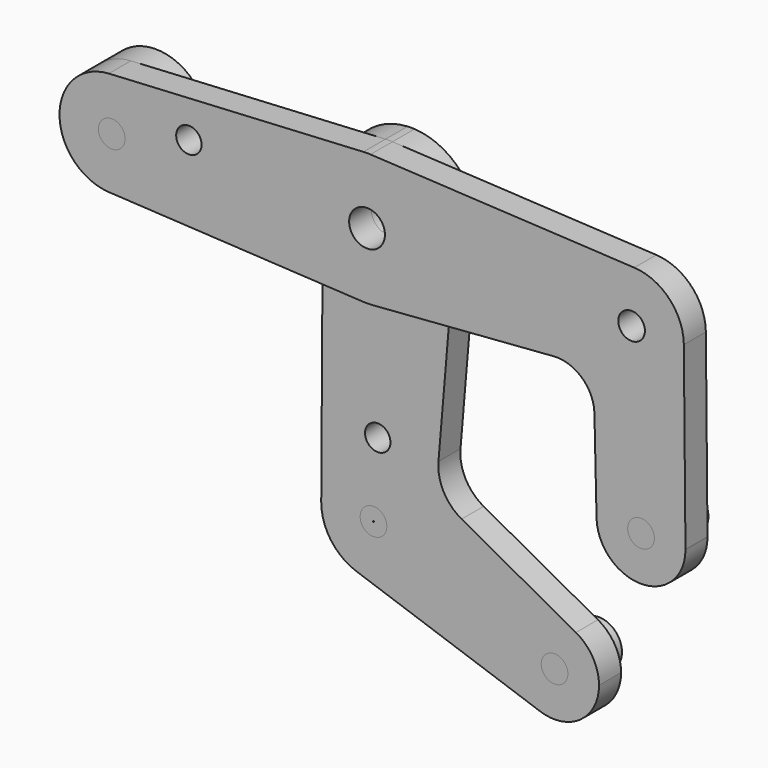
from build123d import *

# Parameters (mm, degrees)
F0_R     = 6.1493367897
F0_R_2   = 5.8576786547
F0_R_3   = 8.2510252631
F1_DEPTH = 12.7
F2_DEPTH = 12.7
F3_R     = 10.7566179169
F5_DEPTH = 25.4
F3_R_2   = 24.0961882632
F4_R     = 24.0590637796
F4_R_2   = 0.2663452523
F4_R_3   = 10.7566179169


with BuildPart() as f1:
    # F0 (on Front) → F1 (new body)
    with BuildSketch(Plane.XZ):
        with BuildLine():
            ThreePointArc((-137.004724496, 53.7728478672), (-144.5318286506, 71.2683255862), (-162.4105469667, 77.8334203262))
            ThreePointArc((-162.4105469667, 77.8334203262), (-185.1971010223, 53.7728478672), (-162.4105469667, 29.7122754082))
            ThreePointArc((-162.4105469667, 29.7122754082), (-144.5318286506, 36.2773701482), (-137.004724496, 53.7728478672))
        make_face()
        with Locations((-161.1009127591, 53.7728478672)):
            Circle(F0_R, mode=Mode.SUBTRACT)
        with BuildLine():
            ThreePointArc((-73.8970993097, 53.9616213386), (-65.4796718147, 74.8089623918), (-45.0619767979, 84.2207871257))
            Line((-45.0619767979, 84.2207871257), (-162.4105469667, 77.8334203262))
            ThreePointArc((-162.4105469667, 77.8334203262), (-144.5318286506, 71.2683255862), (-137.004724496, 53.7728478672))
            ThreePointArc((-137.004724496, 53.7728478672), (-144.5318286506, 36.2773701482), (-162.4105469667, 29.7122754082))
            Line((-162.4105469667, 29.7122754082), (-74.0769888087, 24.9042165128))
            Line((-74.0769888087, 24.9042165128), (-73.8970993097, 53.9616213386))
        make_face()
        with Locations((-125.5404559068, 62.8434497782)):
            Circle(F0_R_2, mode=Mode.SUBTRACT)
        with BuildLine():
            ThreePointArc((-45.0619767979, 23.3249086087), (-65.6094773456, 32.873796427), (-73.8970993097, 53.9616213386))
            Line((-73.8970993097, 53.9616213386), (-74.0769888087, 24.9042165128))
            Line((-74.0769888087, 24.9042165128), (-45.0619767979, 23.3249086087))
        make_face()
        with BuildLine():
            ThreePointArc((-13.0203492827, 51.2005935197), (-12.9388471647, 52.4855731298), (-12.9116636365, 53.7728478672))
            ThreePointArc((-12.9116636365, 53.7728478672), (-21.2847140662, 74.7616793609), (-41.8055673522, 84.2238990469))
            ThreePointArc((-41.8055673522, 84.2238990469), (-43.4338136458, 84.2658439437), (-45.0619767979, 84.2207871257))
            ThreePointArc((-45.0619767979, 84.2207871257), (-65.4796718147, 74.8089623918), (-73.8970993097, 53.9616213386))
            ThreePointArc((-73.8970993097, 53.9616213386), (-65.6094773456, 32.873796427), (-45.0619767979, 23.3249086087))
            ThreePointArc((-45.0619767979, 23.3249086087), (-43.0702384678, 23.2816718981), (-41.0799276521, 23.368584762))
            ThreePointArc((-41.0799276521, 23.368584762), (-21.9308291165, 32.1234215378), (-13.0203492827, 51.2005935197))
        make_face()
        with Locations((-43.4046736365, 53.7728478672)):
            Circle(F0_R_3, mode=Mode.SUBTRACT)
        with BuildLine():
            Line((-15.2090695609, 25.3467012272), (-13.0203492827, 51.2005935197))
            ThreePointArc((-13.0203492827, 51.2005935197), (-21.9308291165, 32.1234215378), (-41.0799276521, 23.368584762))
            Line((-41.0799276521, 23.368584762), (-15.2090695609, 25.3467012272))
        make_face()
        with BuildLine():
            ThreePointArc((-41.8055673522, 84.2238990469), (-21.2847140662, 74.7616793609), (-12.9116636365, 53.7728478672))
            ThreePointArc((-12.9116636365, 53.7728478672), (-12.9388471647, 52.4855731298), (-13.0203492827, 51.2005935197))
            Line((-13.0203492827, 51.2005935197), (-15.2090695609, 25.3467012272))
            Line((-15.2090695609, 25.3467012272), (42.6304365589, 29.7691784017))
            ThreePointArc((42.6304365589, 29.7691784017), (55.6995392523, 25.2975780046), (61.447394796, 12.7373705236))
            Line((61.447394796, 12.7373705236), (62.4270150936, -29.4827839898))
            ThreePointArc((62.4270150936, -29.4827839898), (82.5912356818, -8.509370566), (103.4217411847, -28.8211873993))
            Line((103.4217411847, -28.8211873993), (102.6701248935, 53.9915381907))
            ThreePointArc((102.6701248935, 53.9915381907), (102.6708691973, 53.8821941548), (102.6711173003, 53.7728478672))
            ThreePointArc((102.6711173003, 53.7728478672), (61.0952932065, 37.1870521358), (79.8385749048, 77.8358794288))
            Line((79.8385749048, 77.8358794288), (-41.8055673522, 84.2238990469))
        make_face()
        with BuildLine():
            ThreePointArc((102.6701248935, 53.9915381907), (95.9791200745, 70.4377938061), (79.8385749048, 77.8358794288))
            ThreePointArc((79.8385749048, 77.8358794288), (61.0952932065, 37.1870521358), (102.6711173003, 53.7728478672))
            ThreePointArc((102.6711173003, 53.7728478672), (102.6708691973, 53.8821941548), (102.6701248935, 53.9915381907))
        make_face()
        with Locations((78.5749290371, 53.7728478672)):
            Circle(F0_R, mode=Mode.SUBTRACT)
        with BuildLine():
            ThreePointArc((103.4225855041, -29.0072446459), (103.4223744232, -28.9142150647), (103.4217411847, -28.8211873993))
            ThreePointArc((103.4217411847, -28.8211873993), (82.5912356818, -8.509370566), (62.4270150936, -29.4827839898))
            ThreePointArc((62.4270150936, -29.4827839898), (83.1598278924, -49.506408842), (103.4225855041, -29.0072446459))
        make_face()
        with Locations((82.9220422244, -29.0072446459)):
            Circle(F0_R, mode=Mode.SUBTRACT)
    extrude(amount=F1_DEPTH)


with BuildPart() as f2:
    # F0 (on Front) → F2 (new body)
    with BuildSketch(Plane.XZ):
        with BuildLine():
            ThreePointArc((-13.0203492827, 51.2005935197), (-12.9388471647, 52.4855731298), (-12.9116636365, 53.7728478672))
            ThreePointArc((-12.9116636365, 53.7728478672), (-21.2847140662, 74.7616793609), (-41.8055673522, 84.2238990469))
            ThreePointArc((-41.8055673522, 84.2238990469), (-43.4338136458, 84.2658439437), (-45.0619767979, 84.2207871257))
            ThreePointArc((-45.0619767979, 84.2207871257), (-65.4796718147, 74.8089623918), (-73.8970993097, 53.9616213386))
            ThreePointArc((-73.8970993097, 53.9616213386), (-65.6094773456, 32.873796427), (-45.0619767979, 23.3249086087))
            ThreePointArc((-45.0619767979, 23.3249086087), (-43.0702384678, 23.2816718981), (-41.0799276521, 23.368584762))
            ThreePointArc((-41.0799276521, 23.368584762), (-21.9308291165, 32.1234215378), (-13.0203492827, 51.2005935197))
        make_face()
        with Locations((-43.4046736365, 53.7728478672)):
            Circle(F0_R_3, mode=Mode.SUBTRACT)
        with BuildLine():
            Line((-15.2090695609, 25.3467012272), (-13.0203492827, 51.2005935197))
            ThreePointArc((-13.0203492827, 51.2005935197), (-21.9308291165, 32.1234215378), (-41.0799276521, 23.368584762))
            Line((-41.0799276521, 23.368584762), (-15.2090695609, 25.3467012272))
        make_face()
        with BuildLine():
            ThreePointArc((-45.0619767979, 23.3249086087), (-65.6094773456, 32.873796427), (-73.8970993097, 53.9616213386))
            Line((-73.8970993097, 53.9616213386), (-74.0769888087, 24.9042165128))
            Line((-74.0769888087, 24.9042165128), (-45.0619767979, 23.3249086087))
        make_face()
        with BuildLine():
            Line((-15.2090695609, 25.3467012272), (-41.0799276521, 23.368584762))
            ThreePointArc((-41.0799276521, 23.368584762), (-43.0702384678, 23.2816718981), (-45.0619767979, 23.3249086087))
            Line((-45.0619767979, 23.3249086087), (-74.0769888087, 24.9042165128))
            Line((-74.0769888087, 24.9042165128), (-74.6808307664, -72.6338849963))
            ThreePointArc((-74.6808307664, -72.6338849963), (-50.5105176005, -48.6869847544), (-26.4889159868, -72.7830575806))
            ThreePointArc((-26.4889159868, -72.7830575806), (-36.6048286441, -92.4090144439), (-58.4589669004, -95.5564757645))
            Line((-58.4589669004, -95.5564757645), (26.2038747484, -124.8284797014))
            ThreePointArc((26.2038747484, -124.8284797014), (14.1603031043, -97.1472253354), (42.75710793, -87.4765368913))
            Line((42.75710793, -87.4765368913), (-9.9518053451, -58.5831569567))
            ThreePointArc((-9.9518053451, -58.5831569567), (-18.2433115483, -50.2168226605), (-20.6295718572, -38.6820757448))
            Line((-20.6295718572, -38.6820757448), (-15.2090695609, 25.3467012272))
        make_face()
        with Locations((-48.6188251285, -38.1271646444)):
            Circle(F0_R_2, mode=Mode.SUBTRACT)
        with BuildLine():
            ThreePointArc((-26.4889159868, -72.7830575806), (-50.5105176005, -48.6869847544), (-74.6808307664, -72.6338849963))
            ThreePointArc((-74.6808307664, -72.6338849963), (-70.2542412355, -86.702516588), (-58.4589669004, -95.5564757645))
            ThreePointArc((-58.4589669004, -95.5564757645), (-36.6048286441, -92.4090144439), (-26.4889159868, -72.7830575806))
        make_face()
        with Locations((-50.58510425, -72.7830575806)):
            Circle(F0_R, mode=Mode.SUBTRACT)
        with BuildLine():
            ThreePointArc((53.4033390474, -105.4533221036), (50.542113041, -95.0069466128), (42.75710793, -87.4765368913))
            ThreePointArc((42.75710793, -87.4765368913), (14.1603031043, -97.1472253354), (26.2038747484, -124.8284797014))
            ThreePointArc((26.2038747484, -124.8284797014), (44.7969278184, -122.1506840966), (53.4033390474, -105.4533221036))
        make_face()
        with Locations((32.9027957677, -105.4533221036)):
            Circle(F0_R, mode=Mode.SUBTRACT)
    extrude(amount=-F2_DEPTH)


with BuildPart() as f5:
    # F3 (on face) → F5 (new body)
    with BuildSketch(Plane.XZ.offset(12.7)):
        with Locations((82.9220422244, -29.0072446459)):
            Circle(F3_R)
    extrude(amount=-F5_DEPTH)

    # F6: cut F1, F2
    add(f1.part, mode=Mode.SUBTRACT)
    add(f2.part, mode=Mode.SUBTRACT)


with BuildPart() as f5b:
    # F3 (on face) → F5, piece 2 (new body)
    with BuildSketch(Plane.XZ.offset(12.7)):
        with Locations((-161.1009127591, 53.7728478672)):
            Circle(F3_R_2)
    extrude(amount=-F5_DEPTH)

    # F6: cut F1, F2
    add(f1.part, mode=Mode.SUBTRACT)
    add(f2.part, mode=Mode.SUBTRACT)


with BuildPart() as f5c:
    # F4 (on face) → F5, piece 3 (new body)
    with BuildSketch(Plane.XZ):
        with Locations((-50.58510425, -72.7830575806)):
            Circle(F4_R)
        with Locations((-50.58510425, -72.7830575806)):
            Circle(F4_R_2, mode=Mode.SUBTRACT)
    extrude(amount=-F5_DEPTH)

    # F6: cut F1, F2
    add(f1.part, mode=Mode.SUBTRACT)
    add(f2.part, mode=Mode.SUBTRACT)


with BuildPart() as f5d:
    # F4 (on face) → F5, piece 4 (new body)
    with BuildSketch(Plane.XZ):
        with Locations((32.9027957677, -105.4533221036)):
            Circle(F4_R_3)
    extrude(amount=-F5_DEPTH)

    # F6: cut F1, F2
    add(f1.part, mode=Mode.SUBTRACT)
    add(f2.part, mode=Mode.SUBTRACT)


solid = Compound([f1.part, f2.part, f5.part, f5b.part, f5c.part, f5d.part])
